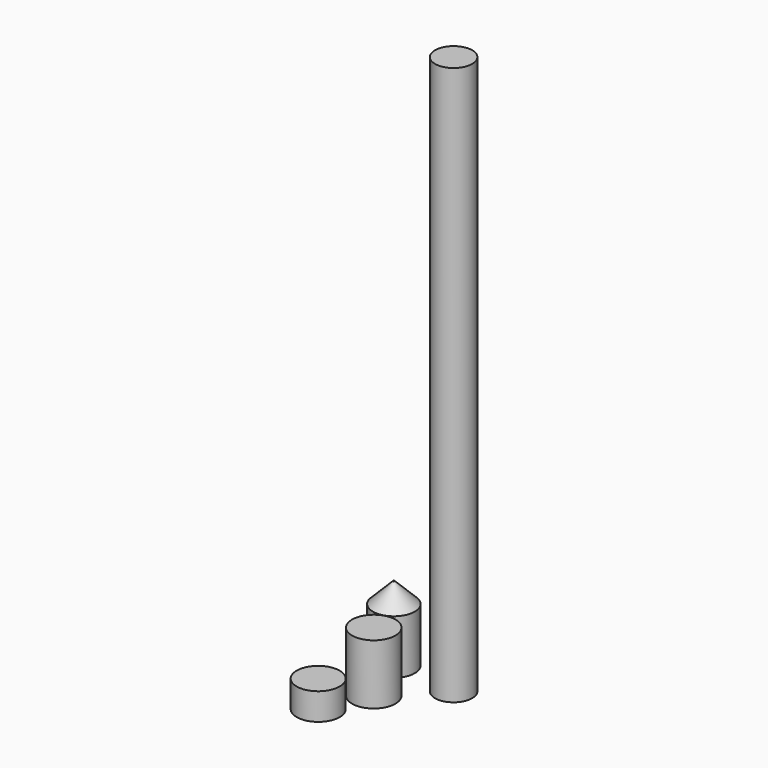
from build123d import *

# Parameters (mm, degrees)
F0_R      = 20.43056521
F1_DEPTH  = 56.5179139376
F4_R      = 19.6707341592
F5_DEPTH  = 70.09729743
F6_SIZE   = 19.05
F7_R      = 20.2538361839
F8_DEPTH  = 25.4
F9_R      = 17.5014397404
F10_DEPTH = 525.8231759071


# Not quite as in the source:
# - the program builds the solid bodies; features that only make, move or delete a surface that nothing else refers to are left out


with BuildPart() as f1:
    # F0 (on Top) → F1 (new body)
    with BuildSketch(Plane.XY):
        with Locations((18.5053218156, 0)):
            Circle(F0_R)
    extrude(amount=F1_DEPTH)


with BuildPart() as f5:
    # F4 (on Top) → F5 (new body)
    with BuildSketch(Plane.XY):
        with Locations((0, 46.7652082443)):
            Circle(F4_R)
    extrude(amount=F5_DEPTH)

    # F6
    f6_edges = [f5.edges().sort_by_distance(p)[0] for p in [
        (-19.670734, 46.765208, 70.097297),
    ]]
    chamfer(f6_edges, length=F6_SIZE)


with BuildPart() as f8:
    # F7 (on Top) → F8 (new body)
    with BuildSketch(Plane.XY):
        with Locations((0, -42.2979965806)):
            Circle(F7_R)
    extrude(amount=F8_DEPTH)


with BuildPart() as f10:
    # F9 (on Top) → F10 (new body)
    with BuildSketch(Plane.XY):
        with Locations((60.0422769785, 42.0709252357)):
            Circle(F9_R)
    extrude(amount=F10_DEPTH)


solid = Compound([f1.part, f5.part, f8.part, f10.part])
